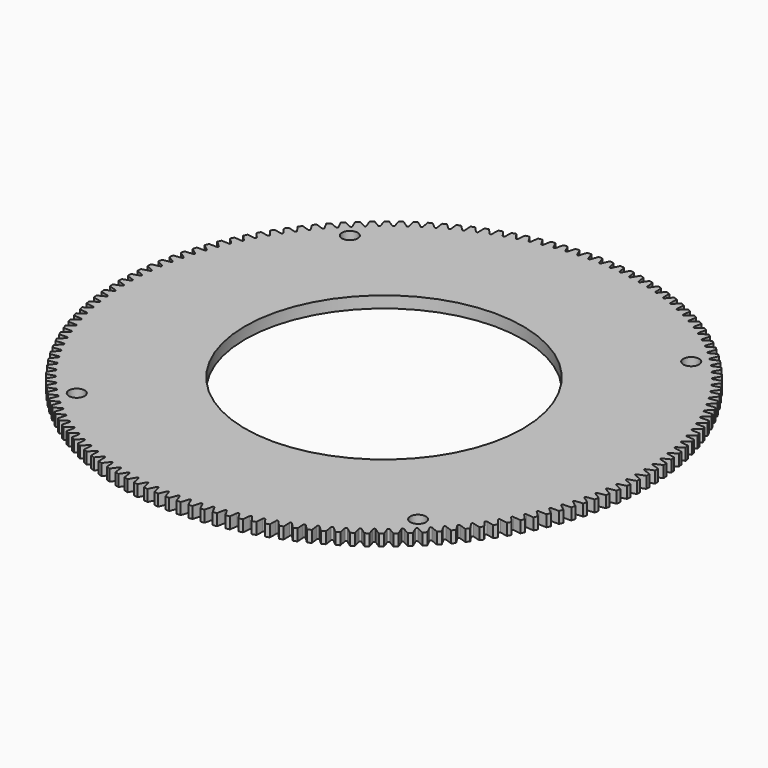
from build123d import *

# Parameters (mm, degrees)
F0_R            = 72.4014057009
F0_R_2          = 2.15265
F0_R_3          = 38.1
F1_DEPTH        = 3.175
F3_DEPTH        = 3.175
F3_COPIES_COUNT = 146


# Not quite as in the source:
# - a pattern or mirror of a feature is missing from the dataset's text; its kind, count and spacing are read off the source's solid


with BuildPart() as f1:
    # F0 (on Top) → F1 (new body)
    with BuildSketch(Plane.XY):
        Circle(F0_R)
        with Locations((-46.83125, -46.83125)):
            Circle(F0_R_2, mode=Mode.SUBTRACT)
        with Locations((46.83125, -46.83125)):
            Circle(F0_R_2, mode=Mode.SUBTRACT)
        with Locations((-46.83125, 46.83125)):
            Circle(F0_R_2, mode=Mode.SUBTRACT)
        Circle(F0_R_3, mode=Mode.SUBTRACT)
        with Locations((46.83125, 46.83125)):
            Circle(F0_R_2, mode=Mode.SUBTRACT)
    extrude(amount=F1_DEPTH)

    # F2 (on face) → F3 (cut, through all)
    with BuildSketch(Plane.XY.offset(3.175)):
        with BuildLine():
            Line((0.2786618065, 70.4227834481), (1.0165388036, 72.3942690848))
            ThreePointArc((1.0165388036, 72.3942690848), (0, 72.4014057009), (-1.0165388036, 72.3942690848))
            Line((-1.0165388036, 72.3942690848), (-0.2786618065, 70.4227834481))
            ThreePointArc((-0.2786618065, 70.4227834481), (0, 70.2295394607), (0.2786618065, 70.4227834481))
        make_face()
    f3 = extrude(amount=-F3_DEPTH, mode=Mode.SUBTRACT)

    # F3_copies: F3 ×146 about axis
    f3_copies_axis = Axis((0, 0, 0), (0, 0, 1))
    for i in range(1, F3_COPIES_COUNT):
        add(f3.rotate(f3_copies_axis, i * 360 / F3_COPIES_COUNT), mode=Mode.SUBTRACT)


solid = f1.part
